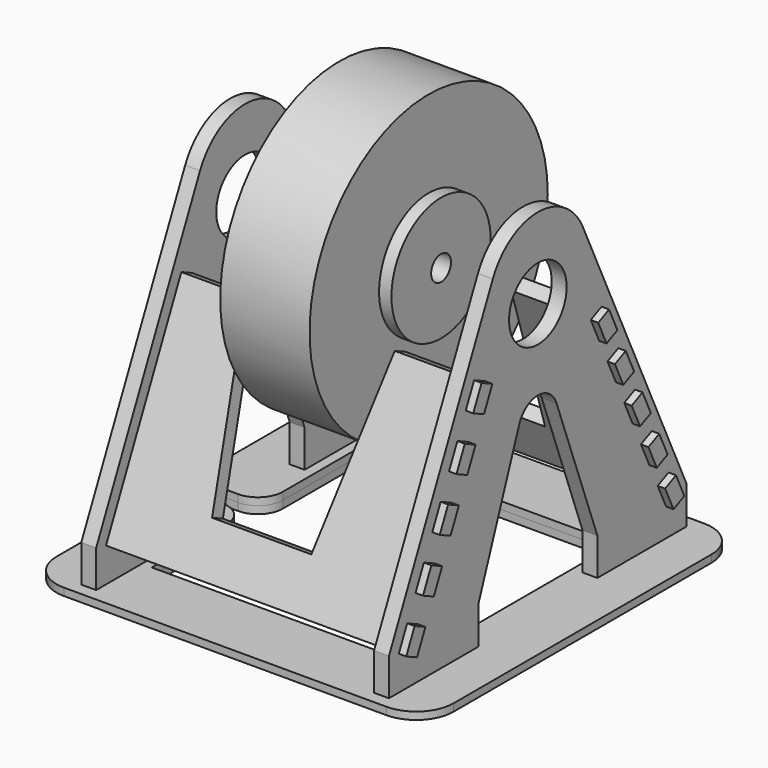
from build123d import *

# Parameters (mm, degrees)
F2_W      = 104
F2_H      = 104
F3_DEPTH  = 3
F4_W      = 160
F4_H      = 160
F4_W_2    = 104
F4_H_2    = 104
F5_DEPTH  = 3
F7_R      = 14.5
F8_DEPTH  = 3
F11_R     = 60
F11_R_2   = 16
F12_DEPTH = 18
F16_DEPTH = 3
F19_W     = 40
F19_H     = 20
F20_DEPTH = 4
F21_R     = 10
F21_2_R   = 10
F22_R     = 15
F23_R     = 5
F24_R     = 25
F24_R_2   = 5
F25_DEPTH = 5


with BuildPart() as f3:
    # F2 (on Top) → F3 (new body)
    with BuildSketch(Plane.XY):
        with BuildLine():
            ThreePointArc((-56, 67), (-63.7781745931, 63.7781745931), (-67, 56))
            Line((-67, 56), (-67, -56))
            ThreePointArc((-67, -56), (-63.7781745931, -63.7781745931), (-56, -67))
            Line((-56, -67), (56, -67))
            ThreePointArc((56, -67), (63.7781745931, -63.7781745931), (67, -56))
            Line((67, -56), (67, 56))
            ThreePointArc((67, 56), (63.7781745931, 63.7781745931), (56, 67))
            Line((56, 67), (-56, 67))
        make_face()
        Rectangle(F2_W, F2_H, mode=Mode.SUBTRACT)
    extrude(amount=-F3_DEPTH)


with BuildPart() as f5:
    # F4 (on Top) → F5 (new body)
    with BuildSketch(Plane.XY):
        Rectangle(F4_W, F4_H)
        Rectangle(F4_W_2, F4_H_2, mode=Mode.SUBTRACT)
    extrude(amount=F5_DEPTH)


with BuildPart() as f8:
    # F7 (on offset) → F8 (new body, symmetric)
    with BuildSketch(Plane.YZ.offset(59)):
        with BuildLine():
            Line((75, 18), (22.6690855497, 130.5409942767))
            ThreePointArc((22.6690855497, 130.5409942767), (0, 145), (-22.6690855497, 130.5409942767))
            Line((-22.6690855497, 130.5409942767), (-75, 18))
            Line((-75, 18), (-75, 3))
            Line((-75, 3), (-60, 3))
            Line((-60, 3), (-60, -5))
            Line((-60, -5), (-54, -5))
            Line((-54, -5), (-54, 3))
            Line((-54, 3), (-48, 3))
            Line((-48, 3), (-48, -5))
            Line((-48, -5), (-42, -5))
            Line((-42, -5), (-42, 3))
            Line((-42, 3), (-36, 3))
            Line((-36, 3), (-36, -5))
            Line((-36, -5), (-30, -5))
            Line((-30, -5), (-30, 3))
            Line((-30, 3), (-30, 18))
            Line((-30, 18), (-9.373248907, 73.4845666771))
            ThreePointArc((-9.373248907, 73.4845666771), (0, 80), (9.373248907, 73.4845666771))
            Line((9.373248907, 73.4845666771), (30, 18))
            Line((30, 18), (30, 3))
            Line((30, 3), (30, -5))
            Line((30, -5), (36, -5))
            Line((36, -5), (36, 3))
            Line((36, 3), (42, 3))
            Line((42, 3), (42, -5))
            Line((42, -5), (48, -5))
            Line((48, -5), (48, 3))
            Line((48, 3), (54, 3))
            Line((54, 3), (54, -5))
            Line((54, -5), (60, -5))
            Line((60, -5), (60, 3))
            Line((60, 3), (75, 3))
            Line((75, 3), (75, 18))
        make_face()
        with Locations((0, 112.5)):
            Circle(F7_R, mode=Mode.SUBTRACT)
    extrude(amount=F8_DEPTH, both=True)


with BuildPart() as f9_1:
    # F9: instance of F8
    add(f8.part.mirror(Plane.YZ))


with BuildPart() as f5_1:
    add(f5.part)

    # F10: cut F9_1, F8
    add(f9_1.part, mode=Mode.SUBTRACT)
    add(f8.part, mode=Mode.SUBTRACT)


with BuildPart() as f3_1:
    add(f3.part)

    # F10: cut F9_1, F8
    add(f9_1.part, mode=Mode.SUBTRACT)
    add(f8.part, mode=Mode.SUBTRACT)


with BuildPart() as f12:
    # F11 (on Right) → F12 (new body, symmetric)
    with BuildSketch(Plane.YZ):
        with Locations((0, 112.5)):
            Circle(F11_R)
        with Locations((0, 112.5)):
            Circle(F11_R_2, mode=Mode.SUBTRACT)
    extrude(amount=F12_DEPTH, both=True)

    # F23
    f23_edges = [f12.edges().sort_by_distance(p)[0] for p in [
        (18, -16, 112.5),
        (-18, -16, 112.5),
    ]]
    fillet(f23_edges, radius=F23_R)


with BuildPart() as f16:
    # F15 (on offset) → F16 (new body, symmetric)
    with BuildSketch(Plane(origin=(0, -61.294280773, 28.5014876938), x_dir=(1, 0, 0), z_dir=(0, -0.906763422, 0.4216397711))):
        Polygon((-65, -4.3012412344), (-65, -14.3012412344), (65, -14.3012412344), (65, -4.3012412344), (56, -4.3012412344), (56, 5.6987587656), (65, 5.6987587656), (65, 15.6987587656), (56, 15.6987587656), (56, 25.6987587656), (65, 25.6987587656), (65, 35.6987587656), (56, 35.6987587656), (56, 45.6987587656), (65, 45.6987587656), (65, 55.6987587656), (56, 55.6987587656), (56, 65.6987587656), (65, 65.6987587656), (65, 75.6987587656), (30, 75.6987587656), (20, 5.6987587656), (-20, 5.6987587656), (-30, 75.6987587656), (-65, 75.6987587656), (-65, 65.6987587656), (-56, 65.6987587656), (-56, 55.6987587656), (-65, 55.6987587656), (-65, 45.6987587656), (-56, 45.6987587656), (-56, 35.6987587656), (-65, 35.6987587656), (-65, 25.6987587656), (-56, 25.6987587656), (-56, 15.6987587656), (-65, 15.6987587656), (-65, 5.6987587656), (-56, 5.6987587656), (-56, -4.3012412344), align=None)
    extrude(amount=F16_DEPTH, both=True)


with BuildPart() as f17_1:
    # F17: instance of F16
    add(f16.part.mirror(Plane.XZ))


with BuildPart() as f9_1_1:
    add(f9_1.part)

    # F18: cut F17_1, F16
    add(f17_1.part, mode=Mode.SUBTRACT)
    add(f16.part, mode=Mode.SUBTRACT)


with BuildPart() as f8_1:
    add(f8.part)

    # F18: cut F17_1, F16
    add(f17_1.part, mode=Mode.SUBTRACT)
    add(f16.part, mode=Mode.SUBTRACT)


with BuildPart() as f20_tool:
    # F19 (on Front) → F20 (new body, symmetric)
    with BuildSketch(Plane.XZ):
        with Locations((-65, 0)):
            Rectangle(F19_W, F19_H)
    extrude(amount=F20_DEPTH, both=True)


with BuildPart() as f3_2:
    add(f3_1.part)

    # F20: cut by f20_tool
    add(f20_tool.part, mode=Mode.SUBTRACT)

    # F21#2
    f21_2_edges = [f3_2.edges().sort_by_distance(p)[0] for p in [
        (-52, 4, -1.5),
        (-52, -4, -1.5),
    ]]
    fillet(f21_2_edges, radius=F21_2_R)


with BuildPart() as f5_2:
    add(f5_1.part)

    # F20: cut by f20_tool
    add(f20_tool.part, mode=Mode.SUBTRACT)

    # F21
    f21_edges = [f5_2.edges().sort_by_distance(p)[0] for p in [
        (-80, 4, 1.5),
        (-80, -4, 1.5),
        (-52, 4, 1.5),
        (-52, -4, 1.5),
    ]]
    fillet(f21_edges, radius=F21_R)

    # F22
    f22_edges = [f5_2.edges().sort_by_distance(p)[0] for p in [
        (-80, -80, 1.5),
        (80, -80, 1.5),
        (80, 80, 1.5),
        (-80, 80, 1.5),
    ]]
    fillet(f22_edges, radius=F22_R)


with BuildPart() as f25:
    # F24 (on face) → F25 (new body, symmetric)
    with BuildSketch(Plane(origin=(-18, 0, 0), x_dir=(0, -1, 0), z_dir=(-1, 0, 0))):
        with Locations((0, 112.5)):
            Circle(F24_R)
        with Locations((0, 112.5)):
            Circle(F24_R_2, mode=Mode.SUBTRACT)
    extrude(amount=F25_DEPTH, both=True)

    # F26: cut F12
    add(f12.part, mode=Mode.SUBTRACT)


with BuildPart() as f27_1:
    # F27: instance of F25
    add(f25.part.mirror(Plane.YZ))


solid = Compound([f12.part, f16.part, f17_1.part, f9_1_1.part, f8_1.part, f3_2.part, f5_2.part, f25.part, f27_1.part])
